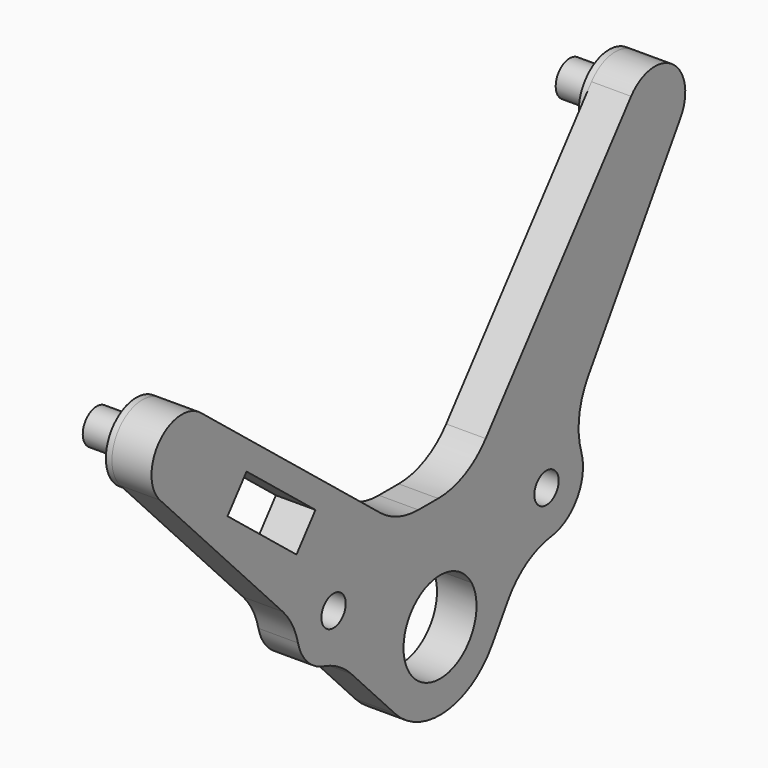
from build123d import *

# Parameters (mm, degrees)
F0_R      = 6
F1_DEPTH  = 5.2
F3_DEPTH  = 5.2
F4_R      = 2
F5_DEPTH  = 5.201
F6_R      = 2.3
F7_DEPTH  = 6
F8_R      = 10
F9_R      = 5
F10_DEPTH = 0.8
F12_DEPTH = 11.201


# Not quite as in the source:
# - after a boolean that leaves OpenCascade's solid faulty, fix() repairs it


with BuildPart() as f1:
    # F0 (on Right) → F1 (new body)
    with BuildSketch(Plane.YZ):
        with BuildLine():
            Line((-46.040940394, 33.401673725), (-7.373073653, -7.0482469386))
            ThreePointArc((-7.373073653, -7.0482469386), (0.98631296, -10.1522010788), (8.5918975137, -5.49720812))
            Line((8.5918975137, -5.49720812), (39.5233468872, 42.8473037055))
            ThreePointArc((39.5233468872, 42.8473037055), (38.2235494383, 49.6065847975), (31.4053950195, 48.6631206432))
            Line((31.4053950195, 48.6631206432), (0, 9.3575391148))
            Line((0, 9.3575391148), (-39.3055815284, 40.7629341343))
            ThreePointArc((-39.3055815284, 40.7629341343), (-46.1155687358, 40.2319246329), (-46.040940394, 33.401673725))
        make_face()
        Circle(F0_R, mode=Mode.SUBTRACT)
    extrude(amount=F1_DEPTH)

    # F2 (on face) → F3 (join, through all)
    with BuildSketch(Plane.YZ.offset(5.2)):
        with BuildLine():
            Line((5.1961524227, 3), (17.5, 3))
            ThreePointArc((17.5, 3), (23.5, 9), (17.5, 15))
            Line((17.5, 15), (-17.5, 15))
            ThreePointArc((-17.5, 15), (-23.5, 9), (-17.5, 3))
            Line((-17.5, 3), (-5.1961524227, 3))
            ThreePointArc((-5.1961524227, 3), (0, 6), (5.1961524227, 3))
        make_face()
    extrude(amount=-F3_DEPTH)

    # F4 (on face) → F5 (cut, through all)
    with BuildSketch(Plane.YZ.offset(5.2)):
        with Locations((-17.5, 9)):
            Circle(F4_R)
        with Locations((17.5, 9)):
            Circle(F4_R)
    extrude(amount=-F5_DEPTH, mode=Mode.SUBTRACT)

    # F6 (on face) → F7 (join)
    with BuildSketch(Plane(origin=(0, 0, 0), x_dir=(0, -1, 0), z_dir=(-1, 0, 0))):
        with Locations((-35.3116324197, 45.5420135683)):
            Circle(F6_R)
        with Locations((42.4266886034, 36.8566967341)):
            Circle(F6_R)
    extrude(amount=F7_DEPTH)

    # F8
    f8_edges = [f1.edges().sort_by_distance(p)[0] for p in [
        (2.6, 4.50836, 15),
        (2.6, -7.061851, 15),
        (2.6, 20.990033, 13.88054),
        (2.6, 14.028522, 3),
        (2.6, -16.978637, 3),
        (2.6, -23.450386, 9.770007),
    ]]
    fillet(f8_edges, radius=F8_R)

    # F9 (on face) → F10 (join)
    with BuildSketch(Plane(origin=(0, 0, 0), x_dir=(0, -1, 0), z_dir=(-1, 0, 0))):
        with Locations((-35.3116324197, 45.5420135683)):
            Circle(F9_R)
        with Locations((42.4266886034, 36.8566967341)):
            Circle(F9_R)
    extrude(amount=F10_DEPTH)

    add(f1.part.fix(), mode=Mode.REPLACE)

    # F11 (on face) → F12 (cut, through all)
    with BuildSketch(Plane.YZ.offset(5.2)):
        Polygon((-20.4751875523, 21.877324197), (-31.8032760129, 30.9285347143), (-34.9243830879, 27.0222973141), (-23.5962946273, 17.9710867968), align=None)
    extrude(amount=-F12_DEPTH, mode=Mode.SUBTRACT)


solid = f1.part
